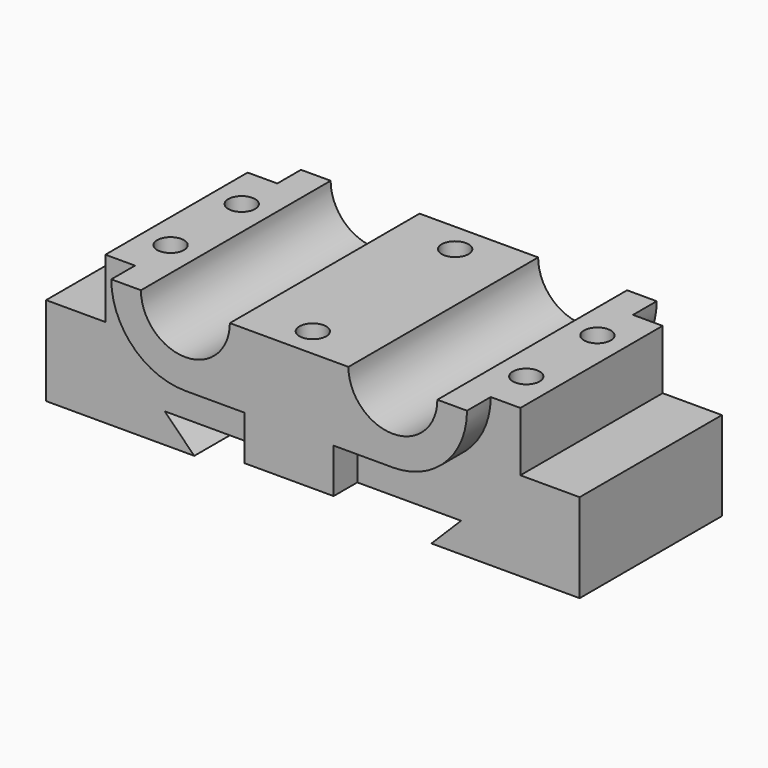
from build123d import *

# Parameters (mm, degrees)
F1_DEPTH         = 38.1
F3_DEPTH         = 12.7
F3_COPIES1_COUNT = 2
F5_DEPTH         = 101.601
F7_D             = 11.5062
F7_DEPTH         = 38.1
F7_TIP           = 3.4568112273
F9_DEPTH         = 101.601


# Not quite as in the source:
# - a pattern or mirror of a feature is missing from the dataset's text; its kind, count and spacing are read off the source's solid


with BuildPart() as f1:
    # F0 (on Front) → F1 (new body, symmetric)
    with BuildSketch(Plane.XZ):
        Polygon((-114.3, 38.1), (-114.3, 0), (114.3, 0), (114.3, 38.1), (88.9, 38.1), (88.9, 63.5), (-88.9, 63.5), (-88.9, 38.1), align=None)
    extrude(amount=F1_DEPTH, both=True)

    # F2 (on face) → F3 (join)
    with BuildSketch(Plane.XZ.offset(38.1)):
        with BuildLine():
            Line((19.05, 31.75), (44.45, 31.75))
            ThreePointArc((44.45, 31.75), (66.9006403027, 41.0493596973), (76.2, 63.5))
            Line((76.2, 63.5), (0, 63.5))
            Line((0, 63.5), (0, 0))
            Line((0, 0), (19.05, 0))
            Line((19.05, 0), (19.05, 31.75))
        make_face()
    f3 = extrude(amount=F3_DEPTH)

    # F3_copies: F3 across plane
    add(f3.mirror(Plane(origin=(0, 0, 0), x_dir=(0, 0, -1), z_dir=(-1, 0, 0))))

    # F3_copies1: F3 ×2 about axis
    f3_copies1_axis = Axis((0, 0, 0), (0, 0, 1))
    for i in range(1, F3_COPIES1_COUNT):
        add(f3.rotate(f3_copies1_axis, i * 360 / F3_COPIES1_COUNT))

    # F3_copies2: F3 across plane
    add(f3.mirror(Plane.ZX))

    # F4 (on face) → F5 (cut, through all)
    with BuildSketch(Plane.XZ.offset(50.8)):
        Polygon((-63.5, 12.7), (-50.8, 0), (50.8, 0), (63.5, 12.7), align=None)
    extrude(amount=-F5_DEPTH, mode=Mode.SUBTRACT)

    # F7
    with Locations(Plane.XY.offset(63.5)):
        with Locations((-76.2, 19.05), (-76.2, -19.05), (0, 38.1), (0, -38.1), (76.2, -19.05), (76.2, 19.05)):
            Hole(F7_D / 2, depth=F7_DEPTH)
            with Locations((0, 0, -(F7_DEPTH + F7_TIP / 2))):  # 118° drill point
                Cone(0, F7_D / 2, F7_TIP, mode=Mode.SUBTRACT)

    # F8 (on face) → F9 (cut, through all)
    with BuildSketch(Plane.XZ.offset(50.8)):
        with BuildLine():
            Line((-25.4, 63.5), (-63.5, 63.5))
            ThreePointArc((-63.5, 63.5), (-44.45, 44.45), (-25.4, 63.5))
        make_face()
        with BuildLine():
            Line((63.5, 63.5), (25.4, 63.5))
            ThreePointArc((25.4, 63.5), (44.45, 44.45), (63.5, 63.5))
        make_face()
    extrude(amount=-F9_DEPTH, mode=Mode.SUBTRACT)


solid = f1.part
